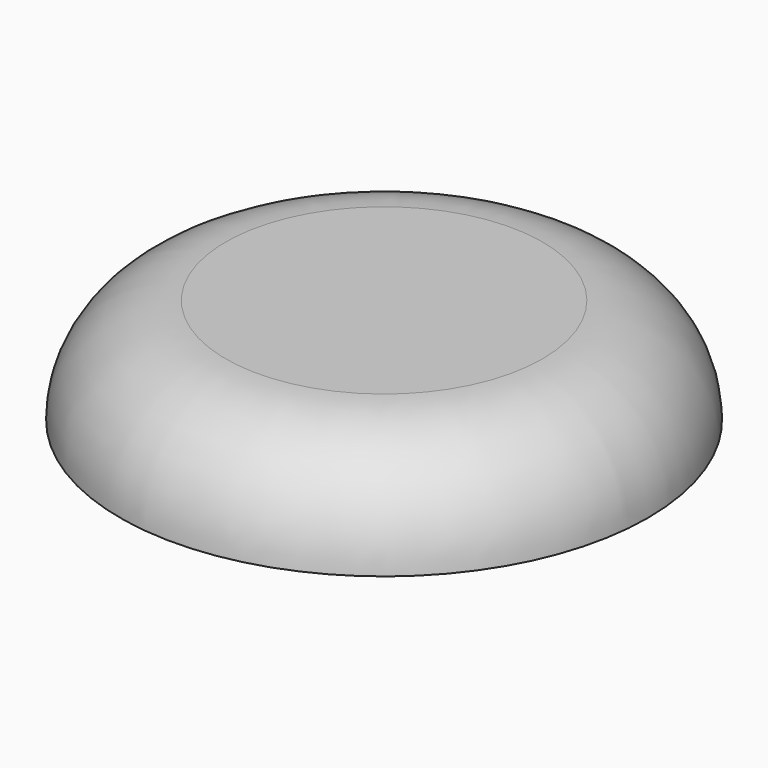
from build123d import *

# Parameters (mm, degrees)
F0_R     = 6.35
F1_DEPTH = 2.54
F2_R     = 2.53999


# Not quite as in the source:
# - a fillet or chamfer is up to 0.001 mm smaller than in the source, because OpenCascade refuses the exact size


with BuildPart() as f1:
    # F0 (on Top) → F1 (new body)
    with BuildSketch(Plane.XY):
        Circle(F0_R)
    extrude(amount=F1_DEPTH)

    # F2 (radius 2.54 in the source; OpenCascade refuses exactly that, so slightly less here)
    f2_edges = [f1.edges().sort_by_distance(p)[0] for p in [
        (-6.35, 0, 2.54),
    ]]
    fillet(f2_edges, radius=F2_R)


solid = f1.part
